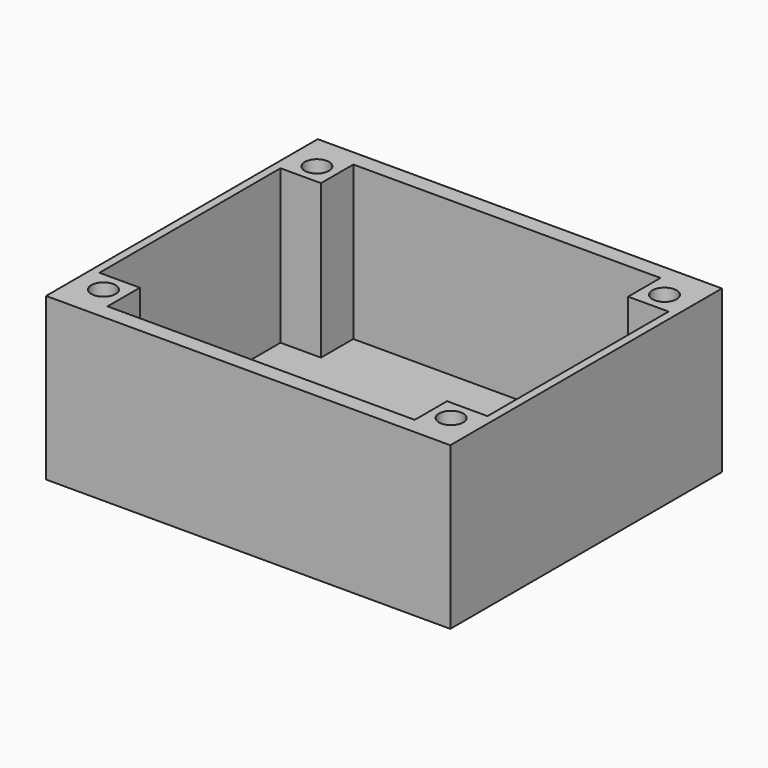
from build123d import *

# Parameters (mm, degrees)
F0_W      = 50
F0_H      = 42
F1_DEPTH  = 20
F2_W      = 38
F2_H      = 38
F3_DEPTH  = 19
F4_W      = 5
F4_H      = 38
F5_DEPTH  = 19
F6_W      = 5
F6_H      = 5
F7_DEPTH  = 19
F8_R      = 1.5
F9_DEPTH  = 10
F10_R     = 2.5
F10_R_2   = 1.5
F11_DEPTH = 5
F12_DEPTH = 1


with BuildPart() as f1:
    # F0 (on Top) → F1 (new body)
    with BuildSketch(Plane.XY):
        with Locations((-37.0541260391, 42.2422697991)):
            Rectangle(F0_W, F0_H)
    extrude(amount=F1_DEPTH)

    # F2 (on face) → F3 (cut)
    with BuildSketch(Plane.XY.offset(20)):
        with Locations((-37.0541260391, 42.2422697991)):
            Rectangle(F2_W, F2_H)
    extrude(amount=-F3_DEPTH, mode=Mode.SUBTRACT)

    # F4 (on face) → F5 (cut)
    with BuildSketch(Plane.XY.offset(20)):
        with Locations((-15.5541260391, 42.2422697991)):
            Rectangle(F4_W, F4_H)
        with Locations((-58.5541260391, 42.2422697991)):
            Rectangle(F4_W, F4_H)
    extrude(amount=-F5_DEPTH, mode=Mode.SUBTRACT)

    # F6 (on face) → F7 (join)
    with BuildSketch(Plane.XY.offset(1)):
        with Locations((-15.5541260391, 58.7422697991)):
            Rectangle(F6_W, F6_H)
        with Locations((-15.5541260391, 25.7422697991)):
            Rectangle(F6_W, F6_H)
        with Locations((-58.5541260391, 58.7422697991)):
            Rectangle(F6_W, F6_H)
        with Locations((-58.5541260391, 25.7422697991)):
            Rectangle(F6_W, F6_H)
    extrude(amount=F7_DEPTH)

    # F8 (on face) → F9 (cut)
    with BuildSketch(Plane.XY.offset(20)):
        with Locations((-15.5541260391, 58.7422697991)):
            Circle(F8_R)
        with Locations((-15.5541260391, 25.7422697991)):
            Circle(F8_R)
        with Locations((-58.5541260391, 25.7422697991)):
            Circle(F8_R)
        with Locations((-58.5541260391, 58.7422697991)):
            Circle(F8_R)
    extrude(amount=-F9_DEPTH, mode=Mode.SUBTRACT)

    # F10 (on face) → F11 (join)
    with BuildSketch(Plane.XY.offset(1)):
        with Locations((-22.0541260391, 57.2422697991)):
            Circle(F10_R)
        with Locations((-22.0541260391, 57.2422697991)):
            Circle(F10_R_2, mode=Mode.SUBTRACT)
        with Locations((-52.0541260391, 27.2422697991)):
            Circle(F10_R)
        with Locations((-52.0541260391, 27.2422697991)):
            Circle(F10_R_2, mode=Mode.SUBTRACT)
    extrude(amount=F11_DEPTH)

    # F12 (cut): faces of the model
    f12_faces = [f1.faces().sort_by_distance(p)[0] for p in [
        (-22.0541260391, 57.2422697991, 1),
        (-52.0541260391, 27.2422697991, 1),
    ]]
    extrude(f12_faces, amount=-F12_DEPTH, mode=Mode.SUBTRACT)


solid = f1.part
